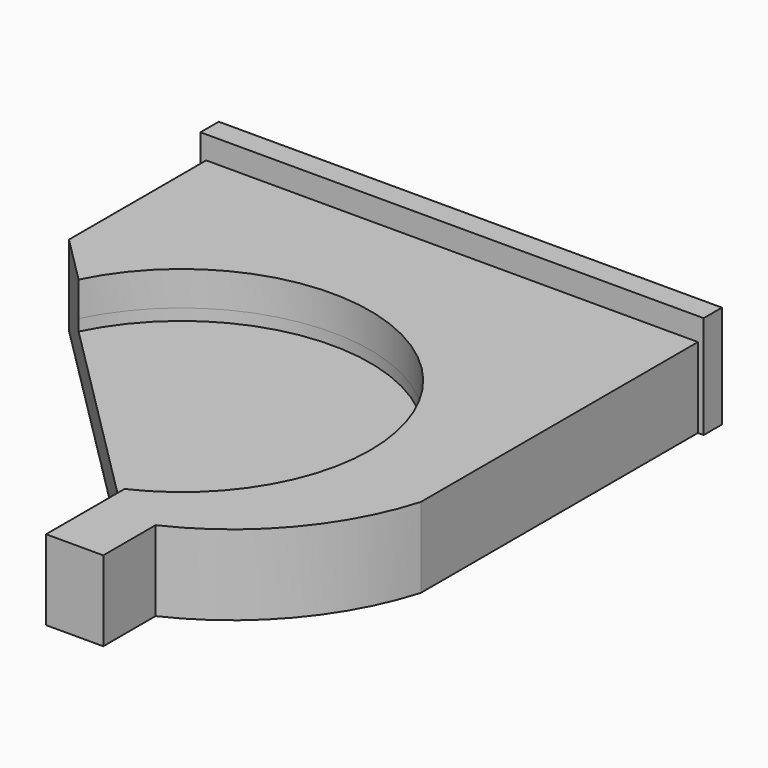
from build123d import *
from build123d import SkipClean  # not in build123d's __all__

# Parameters (mm, degrees)
F1_DEPTH      = 2.5
F1_DEPTH_BACK = 2
F2_DEPTH      = 1.5
F2_DEPTH_BACK = 2
F3_DEPTH      = 2
F4_DEPTH      = 0.5
F5_TEXT_SIZE  = 10.2612590637
F6_DEPTH      = 0.2


# Not quite as in the source:
# - after a boolean that leaves OpenCascade's solid faulty, fix() repairs it
# - Text() gives the source's letters only with a copy of the font that has no kerning and outlines rounded to 1/6400 em; it was checked with that copy


with BuildPart() as f1:
    # F0 (on Top) → F1 (new body, two sides)
    with BuildSketch(Plane.XY) as f1_sk:
        Polygon((11, 13), (0, 13), (-11, 13), (-11, 12), (-10.75, 12), (10.75, 12), (11, 12), align=None)
    extrude(amount=F1_DEPTH)
    extrude(f1_sk.sketch, amount=-F1_DEPTH_BACK)

    # F0 (on Top) → F2 (join, two sides)
    with BuildSketch(Plane.XY) as f2_sk:
        with BuildLine():
            Line((10.75, 12), (-10.75, 12))
            Line((-10.75, 12), (-10.75, 9.5))
            Line((-10.75, 9.5), (-3.1224989992, 9.5))
            ThreePointArc((-3.1224989992, 9.5), (0, 10), (3.1224989992, 9.5))
            Line((3.1224989992, 9.5), (10.75, 9.5))
            Line((10.75, 9.5), (10.75, 12))
        make_face()
        with BuildLine():
            Line((10.75, -3.1428571429), (10.75, 9.5))
            Line((10.75, 9.5), (3.1224989992, 9.5))
            ThreePointArc((3.1224989992, 9.5), (9.9897373659, -0.4529319594), (2.25, -9.743587635))
            Line((2.25, -9.743587635), (2.25, -13))
            Line((2.25, -13), (4.75, -13))
            Line((4.75, -13), (4.75, -10.1428571429))
            ThreePointArc((4.75, -10.1428571429), (8.5036756758, -7.288864865), (10.75, -3.1428571429))
        make_face()
        with BuildLine():
            Line((-3.1224989992, 9.5), (-10.75, 9.5))
            Line((-10.75, 9.5), (-10.75, 4.5))
            Line((-10.75, 4.5), (-9.4680572282, 3.2180572282))
            ThreePointArc((-9.4680572282, 3.2180572282), (-7.0353555543, 7.1066006096), (-3.1224989992, 9.5))
        make_face()
        with BuildLine():
            Line((3.1224989992, 9.5), (-3.1224989992, 9.5))
            ThreePointArc((-3.1224989992, 9.5), (-7.0353555543, 7.1066006096), (-9.4680572282, 3.2180572282))
            Line((-9.4680572282, 3.2180572282), (-8.6448147994, 2.3948147994))
            ThreePointArc((-8.6448147994, 2.3948147994), (-2.5904659048, 6.9008561003), (4.5961940777, 4.5961940777))
            ThreePointArc((4.5961940777, 4.5961940777), (6.3845692761, 1.9197014499), (7.0125631329, -1.2374368671))
            ThreePointArc((7.0125631329, -1.2374368671), (5.720790427, -5.66976954), (2.25, -8.7140861231))
            Line((2.25, -8.7140861231), (2.25, -9.743587635))
            ThreePointArc((2.25, -9.743587635), (9.9897373659, -0.4529319594), (3.1224989992, 9.5))
        make_face()
        with BuildLine():
            ThreePointArc((3.1224989992, 9.5), (0, 10), (-3.1224989992, 9.5))
            Line((-3.1224989992, 9.5), (3.1224989992, 9.5))
        make_face()
    extrude(amount=F2_DEPTH)
    extrude(f2_sk.sketch, amount=-F2_DEPTH_BACK)

    # F0 (on Top) → F3 (join)
    with BuildSketch(Plane.XY):
        with BuildLine():
            ThreePointArc((4.5961940777, 4.5961940777), (-2.5904659048, 6.9008561003), (-8.6448147994, 2.3948147994))
            Line((-8.6448147994, 2.3948147994), (-3.125, -3.125))
            Line((-3.125, -3.125), (4.5961940777, 4.5961940777))
        make_face()
        with BuildLine():
            Line((2.25, -8.5), (2.25, -8.7140861231))
            ThreePointArc((2.25, -8.7140861231), (5.720790427, -5.66976954), (7.0125631329, -1.2374368671))
            ThreePointArc((7.0125631329, -1.2374368671), (6.3845692761, 1.9197014499), (4.5961940777, 4.5961940777))
            Line((4.5961940777, 4.5961940777), (-3.125, -3.125))
            Line((-3.125, -3.125), (2.25, -8.5))
        make_face()
    extrude(amount=-F3_DEPTH)

    # F0 (on Top) → F4 (cut)
    with BuildSketch(Plane.XY):
        with BuildLine():
            ThreePointArc((4.5961940777, 4.5961940777), (-2.5904659048, 6.9008561003), (-8.6448147994, 2.3948147994))
            Line((-8.6448147994, 2.3948147994), (-3.125, -3.125))
            Line((-3.125, -3.125), (4.5961940777, 4.5961940777))
        make_face()
        with BuildLine():
            Line((2.25, -8.5), (2.25, -8.7140861231))
            ThreePointArc((2.25, -8.7140861231), (5.720790427, -5.66976954), (7.0125631329, -1.2374368671))
            ThreePointArc((7.0125631329, -1.2374368671), (6.3845692761, 1.9197014499), (4.5961940777, 4.5961940777))
            Line((4.5961940777, 4.5961940777), (-3.125, -3.125))
            Line((-3.125, -3.125), (2.25, -8.5))
        make_face()
    with SkipClean():  # cleaning this boolean's faces spoils the solid; the shape is the same uncleaned
        extrude(amount=-F4_DEPTH, mode=Mode.SUBTRACT)

    # F5 (on face) → F6 (cut)
    with BuildSketch(Plane(origin=(0, 0, -2), x_dir=(1, 0, 0), z_dir=(0, 0, -1))):
        with Locations((-2.7151571581, -3.853263684)):
            Text('+', F5_TEXT_SIZE, font='Open Sans', font_style=FontStyle.BOLD, text_align=(TextAlign.LEFT, TextAlign.BOTTOM))
    extrude(amount=-F6_DEPTH, mode=Mode.SUBTRACT)

    add(f1.part.fix(), mode=Mode.REPLACE)


solid = f1.part
